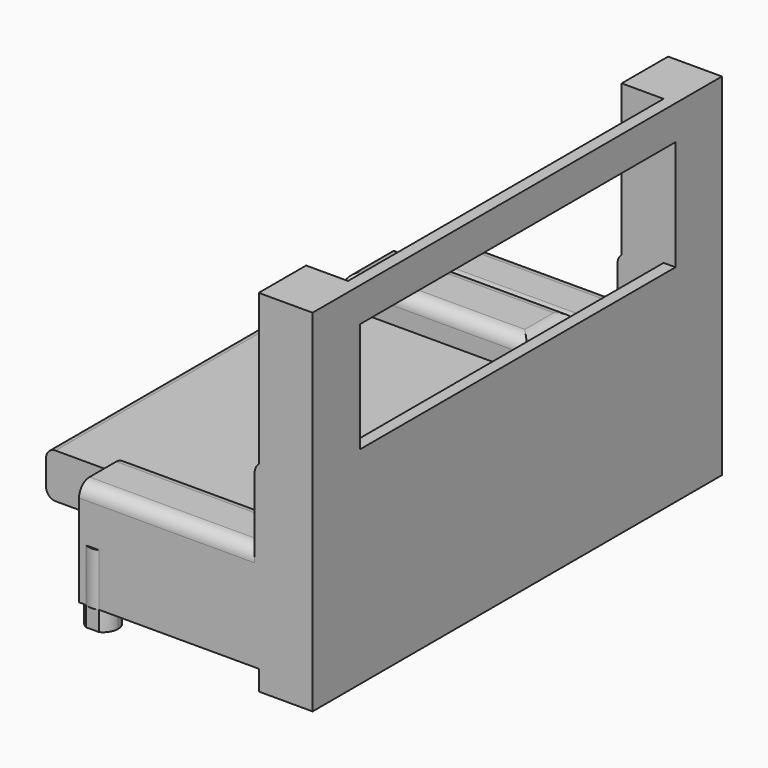
from build123d import *

# Parameters (mm, degrees)
F0_W         = 22.5927522406
F0_H         = 49.5025906712
F1_DEPTH     = 10.16
F2_DEPTH     = 3.81
F3_W         = 11.2244246993
F3_H         = 99.0051813424
F4_DEPTH     = 25.4
F6_DEPTH     = 10.16
F7_R         = 2.54
F8_W         = 33.9610797819
F8_H         = 38.1342638284
F8_H_2       = 37.1269418392
F9_DEPTH     = 5.842
F10_R        = 2.54
F11_W        = 99.0051813424
F11_H        = 67.9221570026
F11_W_2      = 75.9807229042
F11_H_2      = 8.63417238
F12_DEPTH    = 10.414
F13_W        = 19.139082171
F13_H        = 29.1566260799
F13_W_2      = 6.5123029053
F13_H_2      = 0.8140355349
F13_W_3      = 18.2694643736
F13_W_4      = 7.5298482552
F13_W_5      = 18.2365168585
F13_W_6      = 7.1228295565
F13_W_7      = 18.1018151343
F13_W_8      = 7.1228314191
F14_DEPTH    = 0.254
F15_DEPTH    = 1.524
F16_DEPTH    = 60.96
F17_W        = 8.1115535974
F17_H        = 76.3251371682
F17_W_2      = 2.3215521545
F18_DEPTH    = 55.88
F19_R        = 1.8396307345
F20_T4_DEPTH = 85.1788765768
F21_W        = 35.6879150495
F21_H        = 12.0312273502
F22_DEPTH    = 5.842
F23_R        = 2.54
F24_W        = 76.3251371682
F24_H        = 21.320472064
F25_DEPTH    = 25.4


# Not quite as in the source:
# - a fillet or chamfer that OpenCascade refuses, or shapes differently, is made with other operations: its cross-section is extruded or revolved along the edge and cut away or added
# - a feature names something its author has since deleted; it is built from what else it names


with BuildPart() as f1:
    # F0 (on Top) → F1 (new body)
    with BuildSketch(Plane.XY):
        with BuildLine():
            Line((-35.3594812499, 51.6611337662), (-36.6952344775, 51.6611337662))
            Line((-36.6952344775, 51.6611337662), (-36.6952344775, 50.3253805386))
            ThreePointArc((-36.6952344775, 50.3253805386), (-36.1400711383, 51.105970427), (-35.3594812499, 51.6611337662))
        make_face()
        with BuildLine():
            ThreePointArc((-32.8504798068, 51.6611337662), (-34.1049805284, 51.9489325583), (-35.3594812499, 51.6611337662))
            Line((-35.3594812499, 51.6611337662), (-32.8504798068, 51.6611337662))
        make_face()
        with BuildLine():
            Line((-32.8504798068, 51.6611337662), (-35.3594812499, 51.6611337662))
            ThreePointArc((-35.3594812499, 51.6611337662), (-36.1400711383, 51.105970427), (-36.6952344775, 50.3253805386))
            Line((-36.6952344775, 50.3253805386), (-36.6952344775, 47.8163790954))
            ThreePointArc((-36.6952344775, 47.8163790954), (-33.4614356183, 46.2656993361), (-31.2269277871, 49.070879817))
            ThreePointArc((-31.2269277871, 49.070879817), (-31.6663634179, 50.5993869876), (-32.8504798068, 51.6611337662))
        make_face()
        with BuildLine():
            Line((-36.6952344775, 47.8163790954), (-36.6952344775, 50.3253805386))
            ThreePointArc((-36.6952344775, 50.3253805386), (-36.9830332696, 49.070879817), (-36.6952344775, 47.8163790954))
        make_face()
        with BuildLine():
            Line((-14.1024822369, 51.6611337662), (-32.8504798068, 51.6611337662))
            ThreePointArc((-32.8504798068, 51.6611337662), (-31.6663634179, 50.5993869876), (-31.2269277871, 49.070879817))
            ThreePointArc((-31.2269277871, 49.070879817), (-33.4614356183, 46.2656993361), (-36.6952344775, 47.8163790954))
            Line((-36.6952344775, 47.8163790954), (-36.6952344775, 2.158543095))
            Line((-36.6952344775, 2.158543095), (-14.1024822369, 2.158543095))
            Line((-14.1024822369, 2.158543095), (-14.1024822369, 51.6611337662))
        make_face()
        with Locations((-2.8061061166, 26.9098384306)):
            Rectangle(F0_W, F0_H)
        with BuildLine():
            Line((-14.1024822369, 2.158543095), (-36.6952344775, 2.158543095))
            Line((-36.6952344775, 2.158543095), (-36.6952344775, -43.4992929054))
            ThreePointArc((-36.6952344775, -43.4992929054), (-33.4614356183, -41.9486131461), (-31.2269277871, -44.753793627))
            ThreePointArc((-31.2269277871, -44.753793627), (-31.6663634179, -46.2823007976), (-32.8504798068, -47.3440475762))
            Line((-32.8504798068, -47.3440475762), (-14.1024822369, -47.3440475762))
            Line((-14.1024822369, -47.3440475762), (-14.1024822369, 2.158543095))
        make_face()
        with Locations((-2.8061061166, -22.5927522406)):
            Rectangle(F0_W, F0_H)
        with BuildLine():
            ThreePointArc((-31.2269277871, -44.753793627), (-33.4614356183, -41.9486131461), (-36.6952344775, -43.4992929054))
            Line((-36.6952344775, -43.4992929054), (-36.6952344775, -46.0082943486))
            ThreePointArc((-36.6952344775, -46.0082943486), (-36.1400711383, -46.788884237), (-35.3594812499, -47.3440475762))
            Line((-35.3594812499, -47.3440475762), (-32.8504798068, -47.3440475762))
            ThreePointArc((-32.8504798068, -47.3440475762), (-31.6663634179, -46.2823007976), (-31.2269277871, -44.753793627))
        make_face()
        with BuildLine():
            Line((-36.6952344775, -46.0082943486), (-36.6952344775, -43.4992929054))
            ThreePointArc((-36.6952344775, -43.4992929054), (-36.9830332696, -44.753793627), (-36.6952344775, -46.0082943486))
        make_face()
        with BuildLine():
            ThreePointArc((-35.3594812499, -47.3440475762), (-36.1400711383, -46.788884237), (-36.6952344775, -46.0082943486))
            Line((-36.6952344775, -46.0082943486), (-36.6952344775, -47.3440475762))
            Line((-36.6952344775, -47.3440475762), (-35.3594812499, -47.3440475762))
        make_face()
        with BuildLine():
            ThreePointArc((-35.3594812499, -47.3440475762), (-34.1049805284, -47.6318463683), (-32.8504798068, -47.3440475762))
            Line((-32.8504798068, -47.3440475762), (-35.3594812499, -47.3440475762))
        make_face()
    extrude(amount=F1_DEPTH)

    # F0 (on Top) → F2 (join)
    with BuildSketch(Plane.XY):
        with BuildLine():
            Line((-32.8504798068, 51.6611337662), (-35.3594812499, 51.6611337662))
            ThreePointArc((-35.3594812499, 51.6611337662), (-36.1400711383, 51.105970427), (-36.6952344775, 50.3253805386))
            Line((-36.6952344775, 50.3253805386), (-36.6952344775, 47.8163790954))
            ThreePointArc((-36.6952344775, 47.8163790954), (-33.4614356183, 46.2656993361), (-31.2269277871, 49.070879817))
            ThreePointArc((-31.2269277871, 49.070879817), (-31.6663634179, 50.5993869876), (-32.8504798068, 51.6611337662))
        make_face()
        with BuildLine():
            ThreePointArc((-31.2269277871, -44.753793627), (-33.4614356183, -41.9486131461), (-36.6952344775, -43.4992929054))
            Line((-36.6952344775, -43.4992929054), (-36.6952344775, -46.0082943486))
            ThreePointArc((-36.6952344775, -46.0082943486), (-36.1400711383, -46.788884237), (-35.3594812499, -47.3440475762))
            Line((-35.3594812499, -47.3440475762), (-32.8504798068, -47.3440475762))
            ThreePointArc((-32.8504798068, -47.3440475762), (-31.6663634179, -46.2823007976), (-31.2269277871, -44.753793627))
        make_face()
    extrude(amount=-F2_DEPTH)

    # F3 (on face) → F4 (join)
    with BuildSketch(Plane.XY.offset(10.16)):
        with Locations((2.878057654, 2.158543095)):
            Rectangle(F3_W, F3_H)
    extrude(amount=F4_DEPTH)

    # F5 (on face) → F6 (join)
    with BuildSketch(Plane.XY.offset(10.16)):
        Polygon((-2.7341546956, 40.4367111623), (-2.7341546956, 51.6611337662), (-32.8504798068, 51.6611337662), (-35.3594812499, 51.6611337662), (-36.6952344775, 51.6611337662), (-36.6952344775, 50.3253805386), (-36.6952344775, 47.8163790954), (-36.6952344775, 40.4367111623), align=None)
        Polygon((-2.7341546956, -47.3440475762), (-2.7341546956, -35.8318164945), (-36.6952344775, -35.8318164945), (-36.6952344775, -43.4992929054), (-36.6952344775, -46.0082943486), (-36.6952344775, -47.3440475762), (-35.3594812499, -47.3440475762), (-32.8504798068, -47.3440475762), align=None)
    extrude(amount=F6_DEPTH)

    # F7
    f7_edges = [f1.edges().sort_by_distance(p)[0] for p in [
        (-2.734155, 2.158543, 35.56),
        (-19.714695, -35.831816, 20.32),
        (-19.714695, -47.344048, 20.32),
        (-19.714695, 51.661134, 20.32),
        (-19.714695, 40.436711, 20.32),
    ]]
    fillet(f7_edges, radius=F7_R)

    # F8 (on face) → F9 (join)
    with BuildSketch(Plane.XY.offset(10.16)):
        with Locations((-19.7146945866, 21.3695792481)):
            Rectangle(F8_W, F8_H)
        with Locations((-19.7146945866, -17.2683455748)):
            Rectangle(F8_W, F8_H_2)
    extrude(amount=F9_DEPTH)

    # F10
    f10_edges = [f1.edges().sort_by_distance(p)[0] for p in [
        (-19.714695, 1.295125, 16.002),
        (-19.714695, 2.302447, 16.002),
        (-36.695234, -17.268346, 16.002),
        (-36.695234, 21.369579, 16.002),
    ]]
    fillet(f10_edges, radius=F10_R)

    # F11 (on face) → F12 (join)
    with BuildSketch(Plane.YZ.offset(8.4902700037)):
        with Locations((2.158543095, 30.0757006044)):
            Rectangle(F11_W, F11_H)
        with Locations((2.3897327483, 12.2317448258)):
            Rectangle(F11_W_2, F11_H_2, mode=Mode.SUBTRACT)
    extrude(amount=-F12_DEPTH)

    # F13 (on face) → F14 (join)
    with BuildSketch(Plane(origin=(-1.9237299963, 0, 0), x_dir=(0, -1, 0), z_dir=(-1, 0, 0))):
        with Locations((-30.8671663515, 49.4584660657)):
            Rectangle(F13_W, F13_H)
        with Locations((-30.3225759417, 61.080571264)):
            Rectangle(F13_W_2, F13_H_2, mode=Mode.SUBTRACT)
        with Locations((-11.2932752818, 49.4584660657)):
            Rectangle(F13_W_3, F13_H)
        with Locations((-11.4979553036, 61.080571264)):
            Rectangle(F13_W_4, F13_H_2, mode=Mode.SUBTRACT)
        with Locations((7.7183801332, 49.4584660657)):
            Rectangle(F13_W_5, F13_H)
        with Locations((7.9371919855, 61.080571264)):
            Rectangle(F13_W_6, F13_H_2, mode=Mode.SUBTRACT)
        with Locations((26.7809126526, 49.4584660657)):
            Rectangle(F13_W_7, F13_H)
        with Locations((27.0670773461, 61.080571264)):
            Rectangle(F13_W_8, F13_H_2, mode=Mode.SUBTRACT)
    extrude(amount=F14_DEPTH)

    # F13 (on face) → F15 (join)
    with BuildSketch(Plane(origin=(-1.9237299963, 0, 0), x_dir=(0, -1, 0), z_dir=(-1, 0, 0))):
        with Locations((27.0670773461, 61.080571264)):
            Rectangle(F13_W_8, F13_H_2)
        with Locations((7.9371919855, 61.080571264)):
            Rectangle(F13_W_6, F13_H_2)
        with Locations((-11.4979553036, 61.080571264)):
            Rectangle(F13_W_4, F13_H_2)
        with Locations((-30.3225759417, 61.080571264)):
            Rectangle(F13_W_2, F13_H_2)
    extrude(amount=F15_DEPTH)

    # F11 (on face) → F16 (join)
    with BuildSketch(Plane.YZ.offset(8.4902700037)):
        with Locations((2.3897327483, 12.2317448258)):
            Rectangle(F11_W_2, F11_H_2)
    extrude(amount=-F16_DEPTH)

    # F17 (on face) → F18 (cut)
    with BuildSketch(Plane.XY.offset(64.0367791057)):
        with Locations((2.1320468024, 2.274138853)):
            Rectangle(F17_W, F17_H)
        with Locations((-3.0845060736, 2.274138853)):
            Rectangle(F17_W_2, F17_H)
    extrude(amount=-F18_DEPTH, mode=Mode.SUBTRACT)

    # F19
    f19_edges = [f1.edges().sort_by_distance(p)[0] for p in [
        (-52.46973, 2.389733, 16.548831),
        (-52.46973, 2.389733, 7.914659),
    ]]
    fillet(f19_edges, radius=F19_R)

    # F20: fillet of radius 1.8396307345 on 1 edges, made by hand


with BuildPart() as f20_tool2:
    # F20_s3 → F20_t4 (new body)
    with BuildSketch(Plane.XZ.offset(-44.9791710367)):
        with BuildLine():
            ThreePointArc((-6.0849128853, 16.5488310158), (-4.7840975181, 16.0100156486), (-4.2452821508, 14.7092002813))
            Line((-4.2452821508, 14.7092002813), (-4.2452821508, 16.5488310158))
            Line((-4.2452821508, 16.5488310158), (-6.0849128853, 16.5488310158))
        make_face()
    extrude(amount=F20_T4_DEPTH)

    split(bisect_by=Plane.XZ.offset(-40.4367111623), keep=Keep.TOP)

    split(bisect_by=Plane.XZ.offset(35.8318164945), keep=Keep.BOTTOM)


with BuildPart() as f1_1:
    add(f1.part)

    # F20_t1: cut F20_tool2
    add(f20_tool2.part, mode=Mode.SUBTRACT)

    # F21 (on face) → F22 (join)
    with BuildSketch(Plane.XY.offset(16.5488310158)):
        with Locations((-28.3488673158, 34.3644805253)):
            Rectangle(F21_W, F21_H)
    extrude(amount=F22_DEPTH)

    # F23
    f23_edges = [f1_1.edges().sort_by_distance(p)[0] for p in [
        (-10.50491, 34.364481, 22.390831),
        (-28.348867, 28.348867, 22.390831),
        (-46.192825, 34.364481, 22.390831),
        (-28.348867, 40.380094, 22.390831),
    ]]
    fillet(f23_edges, radius=F23_R)

    # F24 (on face) → F25 (cut)
    with BuildSketch(Plane(origin=(6.1878236011, 0, 0), x_dir=(0, -1, 0), z_dir=(-1, 0, 0))):
        with Locations((-2.274138853, 46.7570151377)):
            Rectangle(F24_W, F24_H)
    extrude(amount=-F25_DEPTH, mode=Mode.SUBTRACT)


solid = f1_1.part
